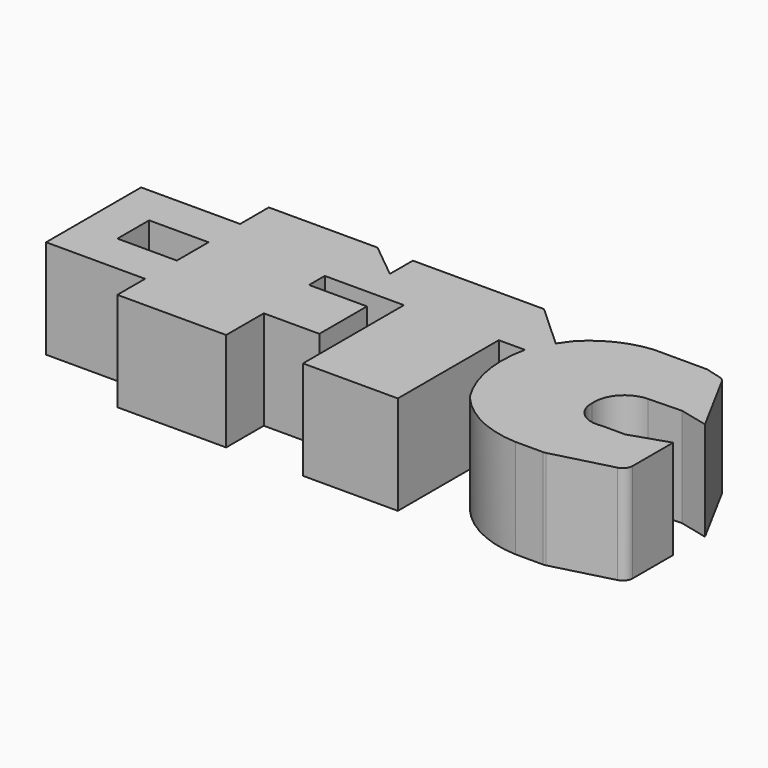
from build123d import *

# Parameters (mm, degrees)
F1_DEPTH = 10
F2_R     = 1
F3_R     = 1
F4_R     = 1
F5_W     = 12
F5_H     = 10
F6_DEPTH = 10
F7_W     = 6
F7_H     = 4
F8_DEPTH = 25


with BuildPart() as f1:
    # F0 (on Top) → F1 (new body)
    with BuildSketch(Plane.XY):
        with BuildLine():
            Line((-11.3350533053, 9.1202929616), (-22.3157362798, 9.1202929616))
            Line((-22.3157362798, 9.1202929616), (-22.3157362798, -10))
            Line((-22.3157362798, -10), (-11.3272070885, -10))
            Line((-11.3272070885, -10), (-11.3272070885, -5.2500292659))
            Line((-11.3272070885, -5.2500292659), (-5.7124928571, -5.2500292659))
            Line((-5.7124928571, -5.2500292659), (-5.7124928571, 0.7569257868))
            Line((-5.7124928571, 0.7569257868), (-11.560020037, 0.7569257868))
            Line((-11.560020037, 0.7569257868), (-11.560020037, 2.7420271654))
            Line((-11.560020037, 2.7420271654), (-3.565690713, 2.7420271654))
            Line((-3.565690713, 2.7420271654), (-3.565690713, -10))
            Line((-3.565690713, -10), (6.0123503208, -10))
            Line((6.0123503208, -10), (6.0123503208, 2.7420271654))
            Line((6.0123503208, 2.7420271654), (8.6545692757, 2.7420271654))
            ThreePointArc((8.6545692757, 2.7420271654), (8.5676927282, -1.911451746), (10.2760922164, -6.2408610247))
            ThreePointArc((10.2760922164, -6.2408610247), (13.6839247097, -8.9288594524), (17.8900292945, -10))
            Line((17.8900292945, -10), (18.7280271202, -10))
            Line((18.7280271202, -10), (20.8180968398, -10))
            Line((20.8180968398, -10), (27.6842637202, -8.2088258604))
            Line((27.6842637202, -8.2088258604), (27.6842637202, -2.3396474093))
            Line((27.6842637202, -2.3396474093), (23.8473247737, -3.5986430012))
            Line((23.8473247737, -3.5986430012), (21.4528143406, -3.5986430012))
            ThreePointArc((21.4528143406, -3.5986430012), (19.3461607597, -3.0392900389), (18.4803195298, -1.038994058))
            ThreePointArc((18.4803195298, -1.038994058), (19.2595578745, 1.248700369), (21.4528143406, 2.2637788206))
            Line((21.4528143406, 2.2637788206), (24.837708557, 2.3617743547))
            Line((24.837708557, 2.3617743547), (27.6842637202, 1.6806415132))
            Line((27.6842637202, 1.6806415132), (27.6842637202, 1.6911900602))
            Line((27.6842637202, 1.6911900602), (23.953304423, 8.5980716969))
            ThreePointArc((23.953304423, 8.5980716969), (22.975945626, 8.8371730757), (22.0104184033, 9.1202929616))
            Line((22.0104184033, 9.1202929616), (16.5817085654, 9.1202929616))
            ThreePointArc((16.5817085654, 9.1202929616), (13.4167991013, 8.2553236841), (10.7552717232, 6.3367054882))
            Line((10.7552717232, 6.3367054882), (9.8750670095, 5.1085127981))
            Line((9.8750670095, 5.1085127981), (5.4812123415, 9.1202929616))
            Line((5.4812123415, 9.1202929616), (-7.7649741434, 9.1202929616))
            Line((-7.7649741434, 9.1202929616), (-7.7649741434, 6.2196037167))
            Line((-7.7649741434, 6.2196037167), (-11.3350533053, 9.1202929616))
        make_face()
    extrude(amount=F1_DEPTH)

    # F2
    f2_edges = [f1.edges().sort_by_distance(p)[0] for p in [
        (23.953304, 8.598072, 5),
        (22.010418, 9.120293, 5),
    ]]
    fillet(f2_edges, radius=F2_R)

    # F3
    f3_edges = [f1.edges().sort_by_distance(p)[0] for p in [
        (17.890029, -10, 5),
        (20.818097, -10, 5),
    ]]
    fillet(f3_edges, radius=F3_R)

    # F4
    f4_edges = [f1.edges().sort_by_distance(p)[0] for p in [
        (27.684264, -8.208826, 5),
        (10.276092, -6.240861, 5),
    ]]
    fillet(f4_edges, radius=F4_R)

    # F5 (on face) → F6 (join)
    with BuildSketch(Plane(origin=(-22.3157362798, 0, 0), x_dir=(0, -1, 0), z_dir=(-1, 0, 0))):
        with Locations((0.5, 5)):
            Rectangle(F5_W, F5_H)
    extrude(amount=F6_DEPTH)

    # F7 (on face) → F8 (cut)
    with BuildSketch(Plane.XY.offset(10)):
        with Locations((-25.3084501922, -0.5)):
            Rectangle(F7_W, F7_H)
    extrude(amount=-F8_DEPTH, mode=Mode.SUBTRACT)


solid = f1.part
